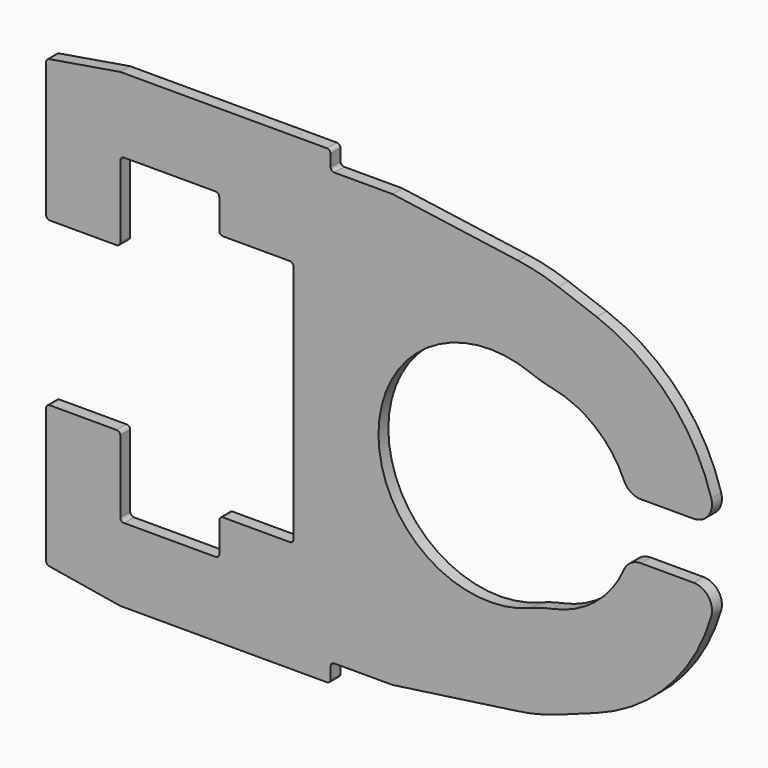
from build123d import *

# Parameters (mm, degrees)
F1_DEPTH = 0.5


# Not quite as in the source:
# - ends of sketch curves that miss each other by under 0.0002 mm in the source are joined


with BuildPart() as f1:
    # F0 (on Front) → F1 (new body, symmetric)
    with BuildSketch(Plane.XZ):
        with BuildLine():
            Line((53.992555, -15.220268), (57.083133, -14.095389))
            ThreePointArc((57.083133, -14.095389), (62.9018568836, -10.252747544), (66.3544503107, -4.1944440905))
            ThreePointArc((66.3544503107, -4.1944440905), (66.1141142416, -2.8747683688), (64.914288, -2.275))
            Line((64.914288, -2.275), (60.670593, -2.275))
            ThreePointArc((60.670593, -2.275), (59.8472095147, -2.5211899521), (59.2941043505, -3.1789471518))
            ThreePointArc((59.2941043505, -3.1789471518), (56.9827494729, -6.2209259886), (53.52425904, -7.8441451998))
            ThreePointArc((53.52425904, -7.8441451998), (52.6431740995, -8.0626756758), (51.7855370008, -8.3602070021))
            ThreePointArc((51.7855370008, -8.3602070021), (39.452831, 0), (51.7855371982, 8.3602074972))
            ThreePointArc((51.7855371982, 8.3602074972), (52.6431743712, 8.0626765952), (53.524259133, 7.844145664))
            ThreePointArc((53.524259133, 7.844145664), (56.9827494729, 6.2209259886), (59.2941043849, 3.1789471667))
            ThreePointArc((59.2941043849, 3.1789471667), (59.8472095147, 2.5211899521), (60.670593, 2.275))
            Line((60.670593, 2.275), (64.914288, 2.275))
            ThreePointArc((64.914288, 2.275), (66.1141145297, 2.8747687527), (66.3544497778, 4.1944449353))
            ThreePointArc((66.3544497778, 4.1944449353), (62.9018565554, 10.2527478944), (57.0831331177, 14.0953893235))
            Line((57.0831331177, 14.0953893235), (53.992555, 15.220268))
            ThreePointArc((53.992555, 15.220268), (52.3736165632, 15.715360306), (50.7118440801, 16.0387645685))
            Line((50.7118440801, 16.0387645685), (40.585713, 17.465))
            Line((40.585713, 17.465), (35.885713, 17.465))
            ThreePointArc((35.885713, 17.465), (35.6735809656, 17.5528679656), (35.585713, 17.765))
            Line((35.585713, 17.765), (35.585713, 18.7))
            ThreePointArc((35.585713, 18.7), (35.4978450344, 18.9121320344), (35.285713, 19))
            Line((35.285713, 19), (18.585713, 19))
            Line((18.585713, 19), (12.836393, 18.04178))
            ThreePointArc((12.836393, 18.04178), (12.656806899, 17.9397743434), (12.585713, 17.745862))
            Line((12.585713, 17.745862), (12.585713, 6.875))
            ThreePointArc((12.585713, 6.875), (12.6735809656, 6.6628679656), (12.885713, 6.575))
            Line((12.885713, 6.575), (18.285713, 6.575))
            ThreePointArc((18.285713, 6.575), (18.4978450344, 6.6628679656), (18.585713, 6.875))
            Line((18.585713, 6.875), (18.585713, 12.7))
            ThreePointArc((18.585713, 12.7), (18.6735809656, 12.9121320344), (18.885713, 13))
            Line((18.885713, 13), (26.285713, 13))
            ThreePointArc((26.285713, 13), (26.4978450344, 12.9121320344), (26.585713, 12.7))
            Line((26.585713, 12.7), (26.585713, 10.3))
            ThreePointArc((26.585713, 10.3), (26.6735809656, 10.0878679656), (26.885713, 10))
            Line((26.885713, 10), (32.285713, 10))
            ThreePointArc((32.285713, 10), (32.4978450344, 9.9121320344), (32.585713, 9.7))
            Line((32.585713, 9.7), (32.585713, -9.7))
            ThreePointArc((32.585713, -9.7), (32.4978450344, -9.9121320344), (32.285713, -10))
            Line((32.285713, -10), (26.885713, -10))
            ThreePointArc((26.885713, -10), (26.6735809656, -10.0878679656), (26.585713, -10.3))
            Line((26.585713, -10.3), (26.585713, -12.7))
            ThreePointArc((26.585713, -12.7), (26.4978450344, -12.9121320344), (26.285713, -13))
            Line((26.285713, -13), (18.885713, -13))
            ThreePointArc((18.885713, -13), (18.6735809656, -12.9121320344), (18.585713, -12.7))
            Line((18.585713, -12.7), (18.585713, -6.875))
            ThreePointArc((18.585713, -6.875), (18.4978450344, -6.6628679656), (18.285713, -6.575))
            Line((18.285713, -6.575), (12.885713, -6.575))
            ThreePointArc((12.885713, -6.575), (12.6735809656, -6.6628679656), (12.585713, -6.875))
            Line((12.585713, -6.875), (12.585713, -17.745862))
            ThreePointArc((12.585713, -17.745862), (12.656806899, -17.9397743434), (12.8363929795, -18.0417801231))
            Line((12.8363929795, -18.0417801231), (18.585713, -19))
            Line((18.585713, -19), (35.285713, -19))
            ThreePointArc((35.285713, -19), (35.4978450344, -18.9121320344), (35.585713, -18.7))
            Line((35.585713, -18.7), (35.585713, -17.765))
            ThreePointArc((35.585713, -17.765), (35.6735809656, -17.5528679656), (35.885713, -17.465))
            Line((35.885713, -17.465), (40.585713, -17.465))
            Line((40.585713, -17.465), (50.711844, -16.038764))
            ThreePointArc((50.711844, -16.038764), (52.3736165632, -15.715360306), (53.992555, -15.220268))
        make_face()
    extrude(amount=F1_DEPTH, both=True)


solid = f1.part
